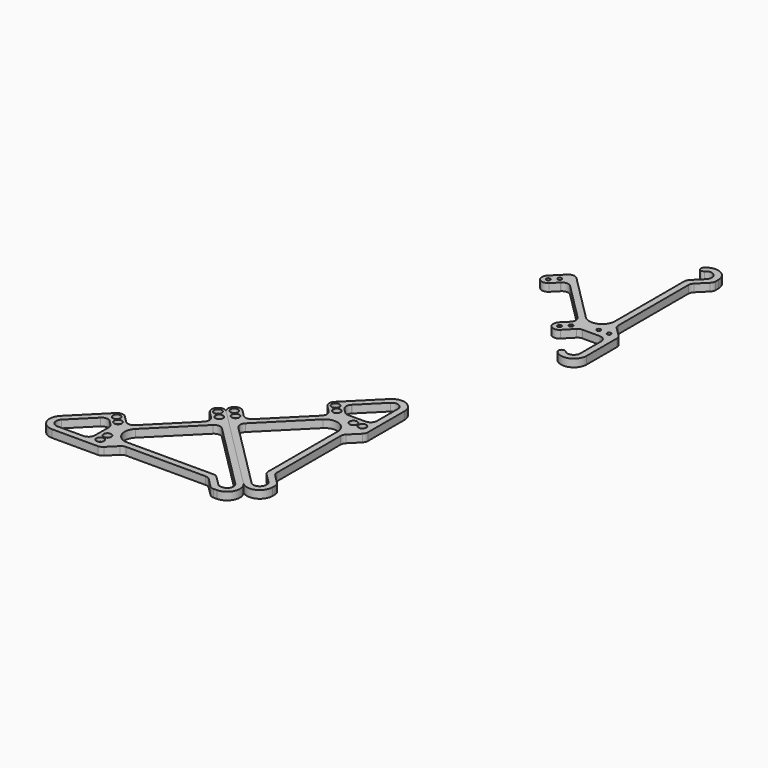
from build123d import *

# Parameters (mm, degrees)
F0_R     = 3
F0_R_2   = 1.5
F1_DEPTH = 6
F2_DEPTH = 3
F4_ANGLE = 180
F5_R     = 3
F5_R_2   = 1.5
F6_DEPTH = 6
F7_DEPTH = 3


# Not quite as in the source:
# - ends of sketch curves that miss each other by under 0.0002 mm in the source are joined
# - a feature names something its author has since deleted; it is built from what else it names


with BuildPart() as f1:
    # F0 (on Top) → F1 (new body)
    with BuildSketch(Plane.XY):
        with BuildLine():
            Line((-44.2507649491, -15.7309638295), (-67.8966558772, -39.3600964056))
            ThreePointArc((-67.8966558772, -39.3600964056), (-70.4563508956, -50.2786340566), (-61.2678443201, -56.7080858167))
            Line((-61.2678443201, -56.7080858167), (-25.6263155519, -56.7080858167))
            ThreePointArc((-25.6263155519, -56.7080858167), (-23.7137171769, -56.3278225468), (-22.0920351666, -55.244872799))
            Line((-22.0920351666, -55.244872799), (-15.0134444525, -48.1712988343))
            ThreePointArc((-15.0134444525, -48.1712988343), (-13.3917624422, -47.0883490865), (-11.4791640672, -46.7080858167))
            Line((-11.4791640672, -46.7080858167), (50.450679434, -46.7080858167))
            ThreePointArc((50.450679434, -46.7080858167), (52.3649153225, -47.0890273668), (53.9874664163, -48.1738054314))
            Line((53.9874664163, -48.1738054314), (61.0510175457, -55.2423662019))
            ThreePointArc((61.0510175457, -55.2423662019), (62.6735686396, -56.3271442665), (64.5878045281, -56.7080858167))
            Line((64.5878045281, -56.7080858167), (67.1692719313, -56.7080858167))
            ThreePointArc((67.1692719313, -56.7080858167), (76.407388831, -50.5365575937), (74.2428458959, -39.6395250461))
            Line((74.2428458959, -39.6395250461), (6.6020689823, 28.0492243407))
            ThreePointArc((6.6020689823, 28.0492243407), (-0.468998363, 28.0517309377), (-0.47150496, 20.9806635924))
            Line((-0.47150496, 20.9806635924), (4.4747450178, 16.0309056146))
            Line((4.4747450178, 16.0309056146), (4.6193445248, 15.8862035542))
            ThreePointArc((4.6193445248, 15.8862035542), (6.0825572283, 12.3501507372), (4.6168379277, 8.8151361866))
            Line((4.6168379277, 8.8151361866), (-25.0928231016, -20.8734689663))
            ThreePointArc((-25.0928231016, -20.8734689663), (-28.6288759187, -22.3366816698), (-32.1638904692, -20.8709623692))
            Line((-32.1638904692, -20.8709623692), (-32.2890579557, -20.7457061109))
            Line((-32.2890579557, -20.7457061109), (-37.0330648079, -15.9937348342))
            ThreePointArc((-37.0330648079, -15.9937348342), (-40.5846985995, -14.2907530076), (-44.2507649491, -15.7309638295))
        make_face()
        with BuildLine():
            ThreePointArc((-61.078326007, -51.6837239265), (-65.6980627371, -48.5963223016), (-64.6126063922, -43.1469369442))
            Line((-64.6126063922, -43.1469369442), (-47.8673994854, -26.413597726))
            Line((-47.8673994854, -26.413597726), (-47.7497701082, -26.2960517153))
            ThreePointArc((-47.7497701082, -26.2960517153), (-44.2137172911, -24.8328390118), (-40.6787027406, -26.2985583124))
            Line((-40.6787027406, -26.2985583124), (-37.2804323511, -29.6992388374))
            ThreePointArc((-37.2804323511, -29.6992388374), (-36.1974826033, -31.3209208476), (-35.8172193334, -33.2335192227))
            Line((-35.8172193334, -33.2335192227), (-35.8172193334, -46.6837239265))
            ThreePointArc((-35.8172193334, -46.6837239265), (-37.2816854275, -50.2192578325), (-40.8172193334, -51.6837239265))
            Line((-40.8172193334, -51.6837239265), (-61.078326007, -51.6837239265))
        make_face(mode=Mode.SUBTRACT)
        with Locations((-29.782678, -49.088475)):
            Circle(F0_R, mode=Mode.SUBTRACT)
        with Locations((-29.782678, -42.088475)):
            Circle(F0_R, mode=Mode.SUBTRACT)
        with Locations((-35.8275559245, -24.2782734668)):
            Circle(F0_R, mode=Mode.SUBTRACT)
        with Locations((-40.7731502233, -19.3243763108)):
            Circle(F0_R, mode=Mode.SUBTRACT)
        with BuildLine():
            ThreePointArc((66.3510826907, -51.7080858167), (64.7719655096, -51.4002516159), (63.4240980576, -50.5218289966))
            Line((63.4240980576, -50.5218289966), (56.0756623135, -43.1681815644))
            ThreePointArc((56.0756623135, -43.1681815644), (54.4531112197, -42.0834034998), (52.5388753312, -41.7024619496))
            Line((52.5388753312, -41.7024619496), (-14.8797955719, -41.7024619496))
            ThreePointArc((-14.8797955719, -41.7024619496), (-23.9809183904, -35.4491639656), (-21.7773304212, -24.628887985))
            Line((-21.7773304212, -24.628887985), (11.6879046534, 8.8126295571))
            ThreePointArc((11.6879046534, 8.8126295571), (15.2239574705, 10.2758422606), (18.758972021, 8.81012296))
            Line((18.758972021, 8.81012296), (70.7040693703, -43.1718151073))
            Line((70.7040693703, -43.1718151073), (70.7045666781, -43.1723127678))
            ThreePointArc((70.7045666781, -43.1723127678), (71.788734305, -48.6213467444), (67.1692719313, -51.7080858167))
            Line((67.1692719313, -51.7080858167), (66.3510826907, -51.7080858167))
        make_face(mode=Mode.SUBTRACT)
        with Locations((8.011532, 19.565186)):
            Circle(F0_R, mode=Mode.SUBTRACT)
        with Locations((3.065282, 24.514944)):
            Circle(F0_R, mode=Mode.SUBTRACT)
        with Locations((-29.782678, -42.088475)):
            Circle(F0_R)
        with Locations((-29.782678, -42.088475)):
            Circle(F0_R_2, mode=Mode.SUBTRACT)
        with Locations((-35.8275559245, -24.2782734668)):
            Circle(F0_R)
        with Locations((-35.8275559245, -24.2782734668)):
            Circle(F0_R_2, mode=Mode.SUBTRACT)
        with Locations((-29.782678, -49.088475)):
            Circle(F0_R)
        with Locations((-29.782678, -49.088475)):
            Circle(F0_R_2, mode=Mode.SUBTRACT)
        with Locations((-40.7731502233, -19.3243763108)):
            Circle(F0_R)
        with Locations((-40.7731502233, -19.3243763108)):
            Circle(F0_R_2, mode=Mode.SUBTRACT)
        with Locations((3.065282, 24.514944)):
            Circle(F0_R)
        with Locations((3.065282, 24.514944)):
            Circle(F0_R_2, mode=Mode.SUBTRACT)
        with Locations((8.011532, 19.565186)):
            Circle(F0_R)
        with Locations((8.011532, 19.565186)):
            Circle(F0_R_2, mode=Mode.SUBTRACT)
    extrude(amount=F1_DEPTH)

    # F0 (on Top) → F2 (cut)
    with BuildSketch(Plane.XY):
        with Locations((8.011532, 19.565186)):
            Circle(F0_R)
        with Locations((8.011532, 19.565186)):
            Circle(F0_R_2, mode=Mode.SUBTRACT)
        with Locations((3.065282, 24.514944)):
            Circle(F0_R)
        with Locations((3.065282, 24.514944)):
            Circle(F0_R_2, mode=Mode.SUBTRACT)
        with Locations((-35.8275559245, -24.2782734668)):
            Circle(F0_R)
        with Locations((-35.8275559245, -24.2782734668)):
            Circle(F0_R_2, mode=Mode.SUBTRACT)
        with Locations((-40.7731502233, -19.3243763108)):
            Circle(F0_R)
        with Locations((-40.7731502233, -19.3243763108)):
            Circle(F0_R_2, mode=Mode.SUBTRACT)
        with Locations((-29.782678, -42.088475)):
            Circle(F0_R)
        with Locations((-29.782678, -42.088475)):
            Circle(F0_R_2, mode=Mode.SUBTRACT)
        with Locations((-29.782678, -49.088475)):
            Circle(F0_R)
        with Locations((-29.782678, -49.088475)):
            Circle(F0_R_2, mode=Mode.SUBTRACT)
    extrude(amount=F2_DEPTH, mode=Mode.SUBTRACT)


with BuildPart() as f3_1:
    # F3: instance of F1
    add(f1.part.mirror(Plane.XY))


with BuildPart() as f1_1:
    # F4: moved
    add(f1.part.rotate(Axis((40.4224574391, -5.7951503527, 0), (0.7068560771, -0.7073573965, 0)), F4_ANGLE))


with BuildPart() as f6:
    # F5 (on Top) → F6 (new body)
    with BuildSketch(Plane.XY):
        with BuildLine():
            ThreePointArc((126.0232128162, 209.5824973705), (122.5654751913, 209.7442884367), (122.2363722776, 206.2984478855))
            ThreePointArc((122.2363722776, 206.2984478855), (133.1549099286, 203.7387528671), (139.5843616887, 212.9272594426))
            Line((139.5843616887, 212.9272594426), (139.5843616887, 242.4152195342))
            ThreePointArc((139.5843616887, 242.4152195342), (139.2040984188, 244.3278179092), (138.121148671, 245.9494999195))
            Line((138.121148671, 245.9494999195), (131.0475747064, 253.0280906336))
            ThreePointArc((131.0475747064, 253.0280906336), (129.9646249585, 254.6497726439), (129.5843616887, 256.5623710189))
            Line((129.5843616887, 256.5623710189), (129.5843616887, 324.6457831967))
            ThreePointArc((129.5843616887, 324.6457831967), (129.9653032388, 326.5600190852), (131.0500813034, 328.182570179))
            Line((131.0500813034, 328.182570179), (138.118642074, 335.2461213084))
            ThreePointArc((138.118642074, 335.2461213084), (139.2034201385, 336.8686724022), (139.5843616887, 338.7829082907))
            Line((139.5843616887, 338.7829082907), (139.5843616887, 341.364375694))
            ThreePointArc((139.5843616887, 341.364375694), (133.4128334657, 350.6024925937), (122.5158009181, 348.4379496586))
            ThreePointArc((122.5158009181, 348.4379496586), (122.5118106204, 344.901670704), (126.0480909444, 344.8991731681))
            Line((126.0480909444, 344.8991731681), (126.0490861253, 344.9001679236))
            ThreePointArc((126.0490861253, 344.9001679236), (131.4979476135, 345.983703449), (134.5843616887, 341.364375694))
            Line((134.5843616887, 341.364375694), (134.5843616887, 340.5461868088))
            ThreePointArc((134.5843616887, 340.5461868088), (134.2765274408, 338.9670695113), (133.3981046937, 337.6192019953))
            Line((133.3981046937, 337.6192019953), (126.0444572615, 330.2707662513))
            ThreePointArc((126.0444572615, 330.2707662513), (124.9596791969, 328.6482151575), (124.5787376467, 326.733979269))
            Line((124.5787376467, 326.733979269), (124.5787376467, 259.3153083659))
            ThreePointArc((124.5787376467, 259.3153083659), (118.3254396627, 250.2141855474), (107.5051636821, 252.4177735166))
            Line((107.5051636821, 252.4177735166), (74.06364614, 285.8830085912))
            Line((74.06364614, 285.8830085912), (70.5293656148, 289.4197957136))
            ThreePointArc((70.5293656148, 289.4197957136), (66.9943510643, 290.8855150141), (63.4582982472, 289.4223023106))
            Line((63.4582982472, 289.4223023106), (54.8270515314, 280.797172745))
            ThreePointArc((54.8270515314, 280.797172745), (54.8245449343, 273.7261053997), (61.8956122796, 273.7235988027))
            Line((61.8956122796, 273.7235988027), (66.8453702574, 278.6698487805))
            Line((66.8453702574, 278.6698487805), (66.9900723178, 278.8144482875))
            ThreePointArc((66.9900723178, 278.8144482875), (70.5261251348, 280.277660991), (74.0611396854, 278.8119416904))
            Line((74.0611396854, 278.8119416904), (103.7497448383, 249.1022806611))
            ThreePointArc((103.7497448383, 249.1022806611), (105.2129575418, 245.566227844), (103.7472382412, 242.0312132935))
            Line((103.7472382412, 242.0312132935), (103.6219819829, 241.906045807))
            Line((103.6219819829, 241.906045807), (98.8700107063, 237.1620389547))
            ThreePointArc((98.8700107063, 237.1620389547), (97.3184058391, 233.604894062), (98.6072397015, 229.9443388136))
            ThreePointArc((98.6072397015, 229.9443388136), (102.2006521828, 228.4213118364), (105.7940646642, 229.9443388136))
            Line((105.7940646642, 229.9443388136), (112.5258589861, 236.8643442339))
            ThreePointArc((112.5258589861, 236.8643442339), (114.1645828984, 237.9839835936), (116.1097950947, 238.3778844293))
            Line((116.1097950947, 238.3778844293), (129.5599997986, 238.3778844293))
            ThreePointArc((129.5599997986, 238.3778844293), (133.0955337045, 236.9134183352), (134.5599997986, 233.3778844293))
            Line((134.5599997986, 233.3778844293), (134.5599997986, 213.1167777557))
            ThreePointArc((134.5599997986, 213.1167777557), (131.4725981736, 208.4970410256), (126.0232128162, 209.5824973705))
        make_face()
        with Locations((102.2006521828, 233.4219535394)):
            Circle(F5_R, mode=Mode.SUBTRACT)
        with Locations((107.1545493389, 238.3675478381)):
            Circle(F5_R, mode=Mode.SUBTRACT)
        with Locations((123.964750872, 244.4124257627)):
            Circle(F5_R, mode=Mode.SUBTRACT)
        with Locations((131.964750872, 244.4124257627)):
            Circle(F5_R, mode=Mode.SUBTRACT)
        with Locations((58.361331872, 277.2603857627)):
            Circle(F5_R, mode=Mode.SUBTRACT)
        with Locations((63.311089872, 282.2066357627)):
            Circle(F5_R, mode=Mode.SUBTRACT)
        with Locations((131.964750872, 244.4124257627)):
            Circle(F5_R)
        with Locations((131.964750872, 244.4124257627)):
            Circle(F5_R_2, mode=Mode.SUBTRACT)
        with Locations((63.311089872, 282.2066357627)):
            Circle(F5_R)
        with Locations((63.311089872, 282.2066357627)):
            Circle(F5_R_2, mode=Mode.SUBTRACT)
        with Locations((58.361331872, 277.2603857627)):
            Circle(F5_R)
        with Locations((58.361331872, 277.2603857627)):
            Circle(F5_R_2, mode=Mode.SUBTRACT)
        with Locations((102.2006521828, 233.4219535394)):
            Circle(F5_R)
        with Locations((102.2006521828, 233.4219535394)):
            Circle(F5_R_2, mode=Mode.SUBTRACT)
        with Locations((107.1545493389, 238.3675478381)):
            Circle(F5_R)
        with Locations((107.1545493389, 238.3675478381)):
            Circle(F5_R_2, mode=Mode.SUBTRACT)
        with Locations((123.964750872, 244.4124257627)):
            Circle(F5_R)
        with Locations((123.964750872, 244.4124257627)):
            Circle(F5_R_2, mode=Mode.SUBTRACT)
    extrude(amount=F6_DEPTH)

    # F5 (on Top) → F7 (cut)
    with BuildSketch(Plane.XY):
        with Locations((58.361331872, 277.2603857627)):
            Circle(F5_R)
        with Locations((58.361331872, 277.2603857627)):
            Circle(F5_R_2, mode=Mode.SUBTRACT)
        with Locations((63.311089872, 282.2066357627)):
            Circle(F5_R)
        with Locations((63.311089872, 282.2066357627)):
            Circle(F5_R_2, mode=Mode.SUBTRACT)
        with Locations((107.1545493389, 238.3675478381)):
            Circle(F5_R)
        with Locations((107.1545493389, 238.3675478381)):
            Circle(F5_R_2, mode=Mode.SUBTRACT)
        with Locations((102.2006521828, 233.4219535394)):
            Circle(F5_R)
        with Locations((102.2006521828, 233.4219535394)):
            Circle(F5_R_2, mode=Mode.SUBTRACT)
        with Locations((123.964750872, 244.4124257627)):
            Circle(F5_R)
        with Locations((123.964750872, 244.4124257627)):
            Circle(F5_R_2, mode=Mode.SUBTRACT)
        with Locations((131.964750872, 244.4124257627)):
            Circle(F5_R)
        with Locations((131.964750872, 244.4124257627)):
            Circle(F5_R_2, mode=Mode.SUBTRACT)
    extrude(amount=F7_DEPTH, mode=Mode.SUBTRACT)


solid = Compound([f3_1.part, f1_1.part, f6.part])
